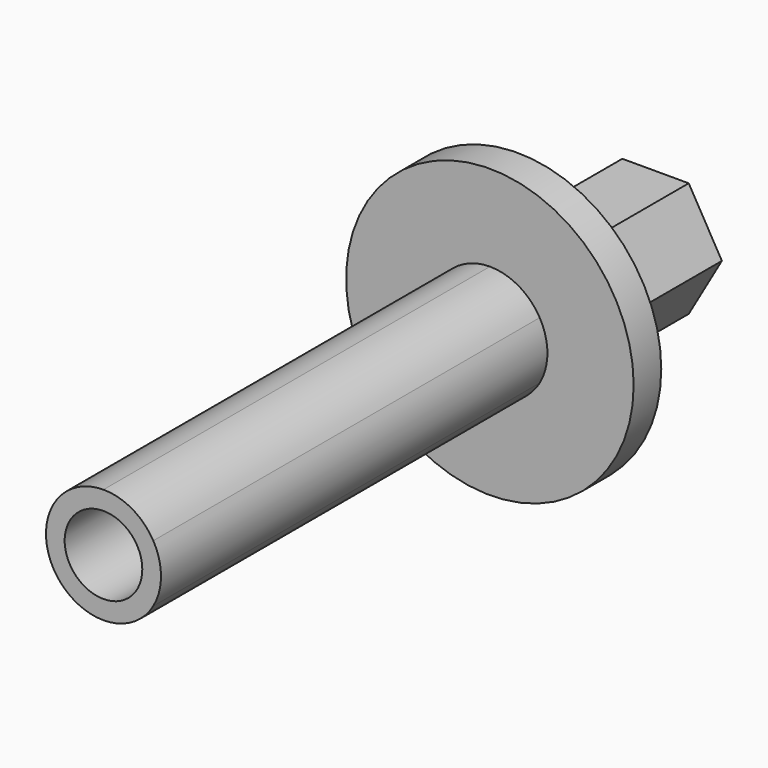
from build123d import *

# Parameters (mm, degrees)
F0_R      = 3.375
F1_DEPTH  = 45
F0_R_2    = 12.5
F2_DEPTH  = 3
F3_DEPTH  = 15
F4_R      = 5
F5_R      = 4.99999
F6_R      = 5
F7_R      = 4.99999
F8_R      = 4.99999
F9_R      = 5
F0_R_3    = 2.5
F10_DEPTH = 15


# Not quite as in the source:
# - a fillet or chamfer is up to 0.001 mm smaller than in the source, because OpenCascade refuses the exact size


with BuildPart() as f1:
    # F0 (on Front) → F1 (new body)
    with BuildSketch(Plane.XZ):
        Polygon((2.8867513459, -5), (5.7735026919, 0), (2.8867513459, 5), (-2.8867513459, 5), (-5.7735026919, 0), (-2.8867513459, -5), align=None)
        Circle(F0_R, mode=Mode.SUBTRACT)
    extrude(amount=F1_DEPTH)

    # F0 (on Front) → F2 (join)
    with BuildSketch(Plane.XZ):
        Circle(F0_R_2)
        Polygon((2.8867513459, 5), (5.7735026919, 0), (2.8867513459, -5), (-2.8867513459, -5), (-5.7735026919, 0), (-2.8867513459, 5), align=None, mode=Mode.SUBTRACT)
        Polygon((2.8867513459, -5), (5.7735026919, 0), (2.8867513459, 5), (-2.8867513459, 5), (-5.7735026919, 0), (-2.8867513459, -5), align=None)
        Circle(F0_R, mode=Mode.SUBTRACT)
    extrude(amount=F2_DEPTH)

    # F4
    f4_edges = [f1.edges().sort_by_distance(p)[0] for p in [
        (2.886751, -24, -5),
    ]]
    fillet(f4_edges, radius=F4_R)

    # F5 (radius 5 in the source; OpenCascade refuses exactly that, so slightly less here)
    f5_edges = [f1.edges().sort_by_distance(p)[0] for p in [
        (-2.886751, -24, -5),
    ]]
    fillet(f5_edges, radius=F5_R)

    # F6
    f6_edges = [f1.edges().sort_by_distance(p)[0] for p in [
        (-5.773503, -24, 0),
    ]]
    fillet(f6_edges, radius=F6_R)

    # F7 (radius 5 in the source; OpenCascade refuses exactly that, so slightly less here)
    f7_edges = [f1.edges().sort_by_distance(p)[0] for p in [
        (-2.886751, -24, 5),
    ]]
    fillet(f7_edges, radius=F7_R)

    # F8 (radius 5 in the source; OpenCascade refuses exactly that, so slightly less here)
    f8_edges = [f1.edges().sort_by_distance(p)[0] for p in [
        (5.773503, -24, 0),
    ]]
    fillet(f8_edges, radius=F8_R)

    # F9
    f9_edges = [f1.edges().sort_by_distance(p)[0] for p in [
        (2.886751, -24, 5),
    ]]
    fillet(f9_edges, radius=F9_R)


with BuildPart() as f3:
    # F0 (on Front) → F3 (new body)
    with BuildSketch(Plane.XZ):
        Polygon((2.8867513459, -5), (5.7735026919, 0), (2.8867513459, 5), (-2.8867513459, 5), (-5.7735026919, 0), (-2.8867513459, -5), align=None)
        Circle(F0_R, mode=Mode.SUBTRACT)
    extrude(amount=-F3_DEPTH)


with BuildPart() as f10:
    # F0 (on Front) → F10 (new body)
    with BuildSketch(Plane.XZ):
        Circle(F0_R)
        Circle(F0_R_3, mode=Mode.SUBTRACT)
    extrude(amount=-F10_DEPTH)


solid = Compound([f1.part, f3.part, f10.part])
